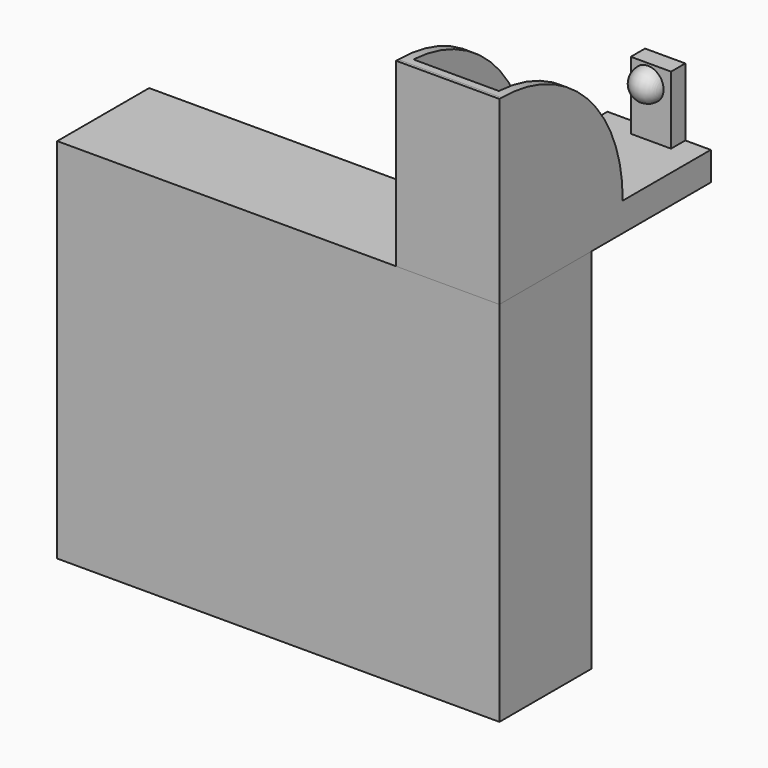
from build123d import *

# Parameters (mm, degrees)
F0_W        = 18
F0_H        = 46
F1_DEPTH    = 5
F2_W        = 18
F2_H        = 1.8357727677
F3_DEPTH    = 26.5
F4_W        = 1.548052609
F4_H        = 26.5
F4_W_2      = 1.5802383423
F5_DEPTH    = 25
F6_T1_DEPTH = 133.3641131145
F6_T3_DEPTH = 133.3962988479
F7_W        = 7.0095323026
F7_H        = 2.1149524208
F7_H_2      = 11.8096721172
F8_DEPTH    = 3.1
F11_W       = 72
F11_H       = 5
F12_DEPTH   = 20
F11_H_2     = 54
F13_DEPTH   = 5.5


# Not quite as in the source:
# - a fillet or chamfer that OpenCascade refuses, or shapes differently, is made with other operations: its cross-section is extruded or revolved along the edge and cut away or added


with BuildPart() as f1:
    # F0 (on Top) → F1 (new body)
    with BuildSketch(Plane.XY):
        with Locations((44.2553941011, 2.0377691388)):
            Rectangle(F0_W, F0_H)
    extrude(amount=F1_DEPTH)

    # F2 (on face) → F3 (join)
    with BuildSketch(Plane.XY.offset(5)):
        with Locations((44.2553941011, -20.0443444774)):
            Rectangle(F2_W, F2_H)
    extrude(amount=F3_DEPTH)

    # F4 (on face) → F5 (join)
    with BuildSketch(Plane(origin=(0, -19.1264580935, 0), x_dir=(-1, 0, 0), z_dir=(0, 1, 0))):
        with Locations((-36.0294204056, 18.25)):
            Rectangle(F4_W, F4_H)
        with Locations((-52.46527493, 18.25)):
            Rectangle(F4_W_2, F4_H)
    extrude(amount=F5_DEPTH)

    # F6: fillet of radius 26.3632121011 on 2 edges, made by hand

    # F6_s2 → F6_t1 (cut)
    with BuildSketch(Plane.YZ.offset(-30.6526361516)):
        with BuildLine():
            ThreePointArc((5.8735419065, 5.1367878989), (-1.8480641441, 23.7783939494), (-20.4896701946, 31.5))
            Line((-20.4896701946, 31.5), (5.8735419065, 31.5))
            Line((5.8735419065, 31.5), (5.8735419065, 5.1367878989))
        make_face()
    extrude(amount=F6_T1_DEPTH, mode=Mode.SUBTRACT)

    # F6_s4 → F6_t3 (cut)
    with BuildSketch(Plane.YZ.offset(-14.2328744939)):
        with BuildLine():
            ThreePointArc((5.8735419065, 5.1367878989), (-1.8480641441, 23.7783939494), (-20.4896701946, 31.5))
            Line((-20.4896701946, 31.5), (5.8735419065, 31.5))
            Line((5.8735419065, 31.5), (5.8735419065, 5.1367878989))
        make_face()
    extrude(amount=F6_T3_DEPTH, mode=Mode.SUBTRACT)

    # F7 (on face) → F8 (join)
    with BuildSketch(Plane(origin=(0, 25.0377691388, 0), x_dir=(-1, 0, 0), z_dir=(0, 1, 0))):
        with Locations((-45.3178305179, 3.9425237896)):
            Rectangle(F7_W, F7_H)
        with Locations((-45.3178305179, 10.9048360586)):
            Rectangle(F7_W, F7_H_2)
    extrude(amount=-F8_DEPTH)

    # F9 (on face) → F10 (revolve)
    with BuildSketch(Plane.XZ.offset(-21.9377691388)):
        with BuildLine():
            ThreePointArc((42.0596776895, 13.6359646723), (44.7758231938, 10.8770558073), (47.5205518922, 13.6075299233))
            ThreePointArc((47.5205518922, 13.6075299233), (47.520514877, 13.6217474905), (47.5204038326, 13.6359646723))
            Line((47.5204038326, 13.6359646723), (42.0596776895, 13.6359646723))
        make_face()
    revolve(axis=Axis((44.790040761, 21.9377691388, 13.6359646723), (1, 0, 0)))


with BuildPart() as f12:
    # F11 (on face) → F12 (new body)
    with BuildSketch(Plane.XZ.offset(20.9622308612)):
        with Locations((12.2553941011, -61.5)):
            Rectangle(F11_W, F11_H)
        Polygon((53.2553941011, -64), (53.2553941011, -5), (48.2553941011, -5), (48.2553941011, -59), (48.2553941011, -64), align=None)
        Polygon((53.2553941011, -5), (53.2553941011, 0), (35.2553941011, 0), (-23.7446058989, 0), (-23.7446058989, -5), (48.2553941011, -5), align=None)
    extrude(amount=-F12_DEPTH)

    # F11 (on face) → F13 (join)
    with BuildSketch(Plane.XZ.offset(20.9622308612)):
        with Locations((12.2553941011, -32)):
            Rectangle(F11_W, F11_H_2)
    extrude(amount=-F13_DEPTH)


solid = Compound([f1.part, f12.part])
